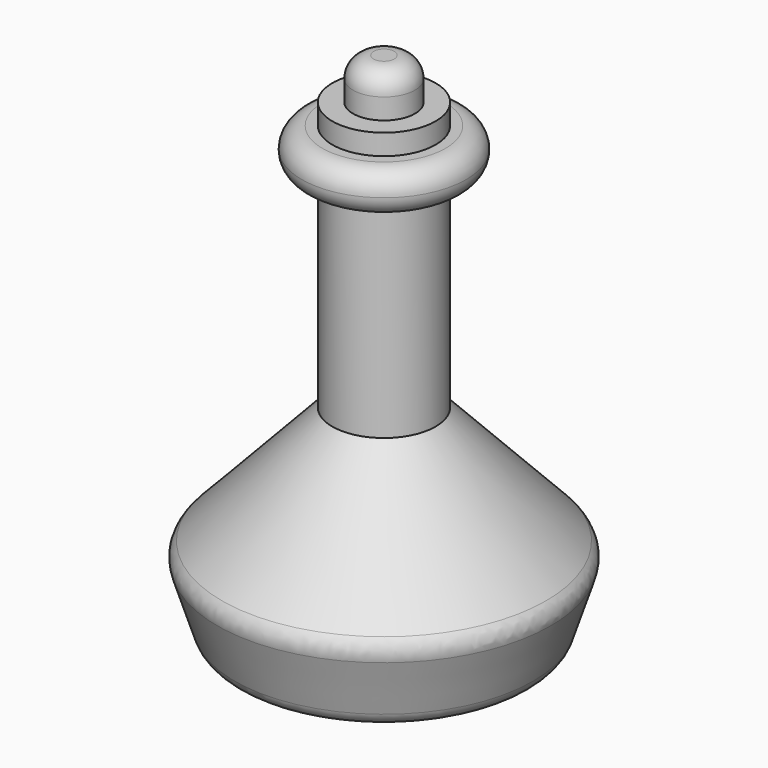
from build123d import *

# Parameters (mm, degrees)
F2_R = 0.2
F3_R = 0.2
F4_R = 0.19999


# Not quite as in the source:
# - a fillet or chamfer is up to 0.001 mm smaller than in the source, because OpenCascade refuses the exact size


with BuildPart() as f1:
    # F0 (on Front) → F1 (revolve)
    with BuildSketch(Plane.XZ):
        Polygon((0, 5), (0, 0), (1.3982689707, 0), (1.6489363067, 0.7781155359), (0.5, 2), (0.5, 4), (0.7954219793, 4), (0.7954219793, 4.4), (0.5, 4.4), (0.5, 4.6), (0.3, 4.6), (0.3, 5), align=None)
    revolve(axis=Axis((0, 0, 2.5), (0, 0, -1)))

    # F2
    f2_edges = [f1.edges().sort_by_distance(p)[0] for p in [
        (-1.398269, 0, 0),
    ]]
    fillet(f2_edges, radius=F2_R)

    # F3
    f3_edges = [f1.edges().sort_by_distance(p)[0] for p in [
        (-1.648936, 0, 0.778116),
        (-0.3, 0, 5),
    ]]
    fillet(f3_edges, radius=F3_R)

    # F4 (radius 0.2 in the source; OpenCascade refuses exactly that, so slightly less here)
    f4_edges = [f1.edges().sort_by_distance(p)[0] for p in [
        (-0.795422, 0, 4.4),
        (-0.795422, 0, 4),
    ]]
    fillet(f4_edges, radius=F4_R)


solid = f1.part
